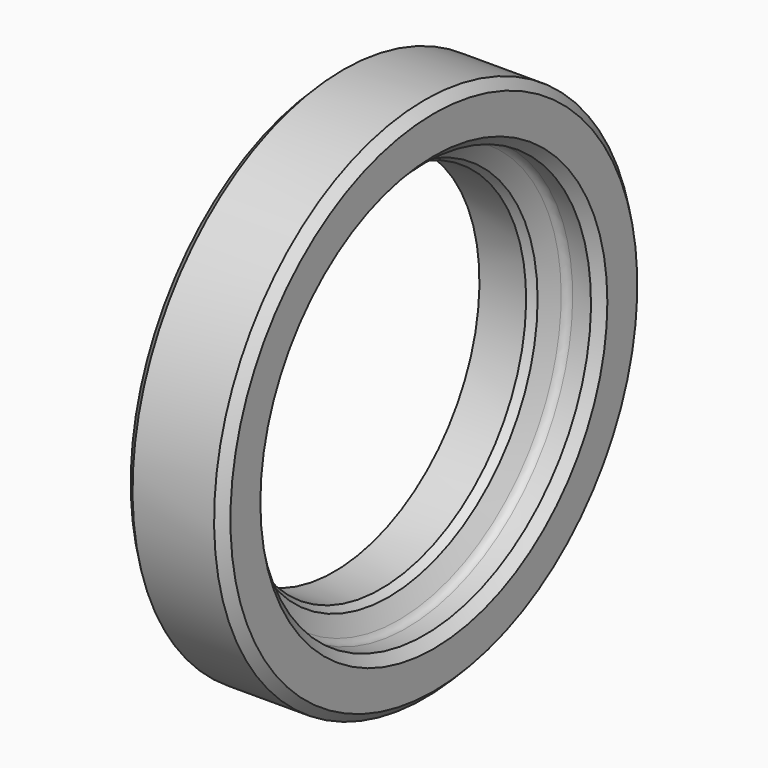
from build123d import *

# Parameters (mm, degrees)
F3_R     = 5
F5_D     = 15
F5_DEPTH = 28.576000561


# Not quite as in the source:
# - a fillet or chamfer that OpenCascade refuses, or shapes differently, is made with other operations: its cross-section is extruded or revolved along the edge and cut away or added


with BuildPart() as f1:
    # F0 (on Front) → F1 (revolve)
    with BuildSketch(Plane.XZ):
        Polygon((26.3250011413, 145), (-27.2249993616, 145), (-28.575000561, 145), (-28.575000561, 100), (0, 100), (8.3250019151, 114.3999986072), (26.3250011413, 114.3999986072), align=None)
    revolve(axis=Axis((-1.3500031339, 0, 0), (1, 0, 0)))

    # F2: chamfer of 5 on 4 edges, made by hand

    # F2_s1 → F2_t2 (revolve, cut)
    with BuildSketch(Plane.XZ):
        Polygon((26.3250011413, 140), (21.3250011413, 145), (26.3250011413, 145), align=None)
    revolve(axis=Axis((26.3250011413, 0, 0), (1, 0, 0)), mode=Mode.SUBTRACT)

    # F2_s3 → F2_t4 (revolve, cut)
    with BuildSketch(Plane.XZ):
        Polygon((21.3250011413, 114.3999986072), (26.3250011413, 119.3999986072), (26.3250011413, 114.3999986072), align=None)
    revolve(axis=Axis((26.3250011413, 0, 0), (1, 0, 0)), mode=Mode.SUBTRACT)

    # F2_s5 → F2_t6 (revolve, cut)
    with BuildSketch(Plane.XZ):
        Polygon((-2.8848150214, 100), (1.4438587798, 102.4974846409), (0, 100), align=None)
    revolve(axis=Axis((0, 0, 0), (1, 0, 0)), mode=Mode.SUBTRACT)

    # F2_s7 → F2_t8 (revolve, cut)
    with BuildSketch(Plane.XZ):
        Polygon((-23.575000561, 145), (-28.575000561, 140), (-28.575000561, 145), align=None)
    revolve(axis=Axis((-28.575000561, 0, 0), (1, 0, 0)), mode=Mode.SUBTRACT)

    # F3
    f3_edges = [f1.edges().sort_by_distance(p)[0] for p in [
        (8.325002, 0, -114.399999),
    ]]
    fillet(f3_edges, radius=F3_R)

    # F5 (through all, one way)
    with BuildSketch(Plane.YZ):
        with Locations((0, 130.4700821638)):
            Circle(F5_D / 2)
    extrude(amount=-F5_DEPTH, mode=Mode.SUBTRACT)


solid = f1.part
